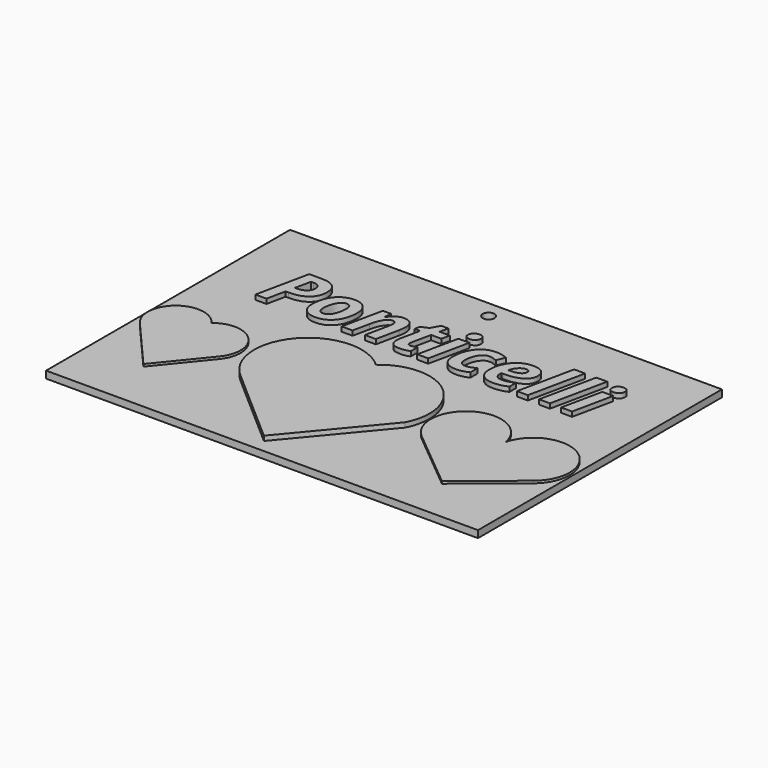
from build123d import *

# Parameters (mm, degrees)
F0_TEXT_SIZE = 31.6076549805
F1_DEPTH     = 5
F0_W         = 183.1867024302
F0_H         = 129.334770143
F2_DEPTH     = 3
F4_DEPTH     = 1
F5_D         = 5


# Not quite as in the source:
# - Text() gives the source's letters only with a copy of the font that has no kerning and outlines rounded to 1/6400 em; it was checked with that copy


with BuildPart() as f1:
    # F0 (on Top) → F1 (new body)
    with BuildSketch(Plane.XY):
        with Locations((-77.6233896613, 8.2242488861)):
            Text('Ponticelli', F0_TEXT_SIZE, font='Open Sans', font_style=FontStyle.BOLDITALIC, text_align=(TextAlign.LEFT, TextAlign.BOTTOM))
        with BuildLine():
            ThreePointArc((19.1414519703, -32.36814572), (13.3379238133, -5.4645873951), (-14.1757235594, -6.1585599173))
            ThreePointArc((-14.1757235594, -6.1585599173), (-46.727283961, -7.8440457742), (-44.2183457938, -40.3425099906))
            Line((-44.2183457938, -40.3425099906), (-11.378755793, -69.0611600876))
            Line((-11.378755793, -69.0611600876), (19.1414519703, -32.36814572))
        make_face()
    extrude(amount=F1_DEPTH)

    # F0 (on Top) → F2 (join)
    with BuildSketch(Plane.XY):
        with Locations((-7.6609440148, -10.0268237293)):
            Rectangle(F0_W, F0_H)
        with BuildLine():
            ThreePointArc((-44.2183457938, -40.3425099906), (-46.727283961, -7.8440457742), (-14.1757235594, -6.1585599173))
            ThreePointArc((-14.1757235594, -6.1585599173), (13.3379238133, -5.4645873951), (19.1414519703, -32.36814572))
            Line((19.1414519703, -32.36814572), (-11.378755793, -69.0611600876))
            Line((-11.378755793, -69.0611600876), (-44.2183457938, -40.3425099906))
        make_face(mode=Mode.SUBTRACT)
        with BuildLine():
            add(Edge.make_bspline(
                [(-61.1701236351, 29.1445655263), (-59.2563789, 27.4999797281), (-59.2563789, 24.2157468278)],
                knots=[0, 0, 0, 1, 1, 1], degree=2))
            add(Edge.make_bspline(
                [(-59.2563789, 24.2157468278), (-59.2563789, 20.4919699754), (-61.8738878281, 18.3708000045)],
                knots=[0, 0, 0, 1, 1, 1], degree=2))
            add(Edge.make_bspline(
                [(-61.8738878281, 18.3708000045), (-64.4913967561, 16.2496300335), (-69.0893228166, 16.2496300335)],
                knots=[0, 0, 0, 1, 1, 1], degree=2))
            Line((-69.0893228166, 16.2496300335), (-70.417832065, 16.2496300335))
            Line((-70.417832065, 16.2496300335), (-72.0969887358, 8.2242488861))
            Line((-72.0969887358, 8.2242488861), (-76.8035661103, 8.2242488861))
            Line((-76.8035661103, 8.2242488861), (-72.0377243827, 30.7891513245))
            Line((-72.0377243827, 30.7891513245), (-66.8175226149, 30.7891513245))
            add(Edge.make_bspline(
                [(-66.8175226149, 30.7891513245), (-63.0838683703, 30.7891513245), (-61.1701236351, 29.1445655263)],
                knots=[0, 0, 0, 1, 1, 1], degree=2))
        make_face(mode=Mode.SUBTRACT)
        with BuildLine():
            add(Edge.make_bspline(
                [(-43.9439516708, 23.9811587635), (-42.1833065144, 22.1612492541), (-42.1833065144, 18.9659128834)],
                knots=[0, 0, 0, 1, 1, 1], degree=2))
            add(Edge.make_bspline(
                [(-42.1833065144, 18.9659128834), (-42.1833065144, 15.7113121596), (-43.2722890024, 13.1950465014)],
                knots=[0, 0, 0, 1, 1, 1], degree=2))
            add(Edge.make_bspline(
                [(-43.2722890024, 13.1950465014), (-44.3612714904, 10.6787808432), (-46.4132997161, 9.2959459378)],
                knots=[0, 0, 0, 1, 1, 1], degree=2))
            add(Edge.make_bspline(
                [(-46.4132997161, 9.2959459378), (-48.4653279418, 7.9131110324), (-51.2902621057, 7.9131110324)],
                knots=[0, 0, 0, 1, 1, 1], degree=2))
            add(Edge.make_bspline(
                [(-51.2902621057, 7.9131110324), (-54.302866721, 7.9131110324), (-56.100552098, 9.7280818457)],
                knots=[0, 0, 0, 1, 1, 1], degree=2))
            add(Edge.make_bspline(
                [(-56.100552098, 9.7280818457), (-57.8982374751, 11.5430526591), (-57.8982374751, 14.5507185783)],
                knots=[0, 0, 0, 1, 1, 1], degree=2))
            add(Edge.make_bspline(
                [(-57.8982374751, 14.5507185783), (-57.8982374751, 17.8398901747), (-56.7944388988, 20.4104814899)],
                knots=[0, 0, 0, 1, 1, 1], degree=2))
            add(Edge.make_bspline(
                [(-56.7944388988, 20.4104814899), (-55.6906403225, 22.9810728051), (-53.6065105722, 24.391070539)],
                knots=[0, 0, 0, 1, 1, 1], degree=2))
            add(Edge.make_bspline(
                [(-53.6065105722, 24.391070539), (-51.522380822, 25.8010682729), (-48.7270788346, 25.8010682729)],
                knots=[0, 0, 0, 1, 1, 1], degree=2))
            add(Edge.make_bspline(
                [(-48.7270788346, 25.8010682729), (-45.7045968271, 25.8010682729), (-43.9439516708, 23.9811587635)],
                knots=[0, 0, 0, 1, 1, 1], degree=2))
        make_face(mode=Mode.SUBTRACT)
        with BuildLine():
            Line((-23.6631961743, 18.0571928027), (-25.717693748, 8.2242488861))
            Line((-25.717693748, 8.2242488861), (-30.3600680733, 8.2242488861))
            Line((-30.3600680733, 8.2242488861), (-28.2463061465, 18.3041276072))
            add(Edge.make_bspline(
                [(-28.2463061465, 18.3041276072), (-27.9993713419, 19.3511311785), (-27.9993713419, 20.141322553)],
                knots=[0, 0, 0, 1, 1, 1], degree=2))
            add(Edge.make_bspline(
                [(-27.9993713419, 20.141322553), (-27.9993713419, 22.0377818518), (-29.6686506206, 22.0377818518)],
                knots=[0, 0, 0, 1, 1, 1], degree=2))
            add(Edge.make_bspline(
                [(-29.6686506206, 22.0377818518), (-31.0860563986, 22.0377818518), (-32.2441806319, 20.2771366955)],
                knots=[0, 0, 0, 1, 1, 1], degree=2))
            add(Edge.make_bspline(
                [(-32.2441806319, 20.2771366955), (-33.4023048652, 18.5164915391), (-34.0640901413, 15.3705421294)],
                knots=[0, 0, 0, 1, 1, 1], degree=2))
            Line((-34.0640901413, 15.3705421294), (-35.5802698412, 8.2242488861))
            Line((-35.5802698412, 8.2242488861), (-40.2226441664, 8.2242488861))
            Line((-40.2226441664, 8.2242488861), (-36.5680090593, 25.480053027))
            Line((-36.5680090593, 25.480053027), (-33.0170865701, 25.480053027))
            Line((-33.0170865701, 25.480053027), (-33.3430405121, 22.2847166563))
            Line((-33.3430405121, 22.2847166563), (-33.2492052864, 22.2847166563))
            add(Edge.make_bspline(
                [(-33.2492052864, 22.2847166563), (-30.997159869, 25.8010682729), (-27.7672526257, 25.8010682729)],
                knots=[0, 0, 0, 1, 1, 1], degree=2))
            add(Edge.make_bspline(
                [(-27.7672526257, 25.8010682729), (-25.6386746106, 25.8010682729), (-24.4731423332, 24.5145379413)],
                knots=[0, 0, 0, 1, 1, 1], degree=2))
            add(Edge.make_bspline(
                [(-24.4731423332, 24.5145379413), (-23.3076100558, 23.2280076097), (-23.3076100558, 20.8327400057)],
                knots=[0, 0, 0, 1, 1, 1], degree=2))
            add(Edge.make_bspline(
                [(-23.3076100558, 20.8327400057), (-23.3076100558, 19.706717297), (-23.6631961743, 18.0571928027)],
                knots=[0, 0, 0, 1, 1, 1], degree=2))
        make_face(mode=Mode.SUBTRACT)
        with BuildLine():
            add(Edge.make_bspline(
                [(-15.1291293296, 12.8073588583), (-15.1291293296, 11.6665200613), (-13.7709879046, 11.6665200613)],
                knots=[0, 0, 0, 1, 1, 1], degree=2))
            add(Edge.make_bspline(
                [(-13.7709879046, 11.6665200613), (-12.7684325982, 11.6665200613), (-11.2670689867, 12.2048379352)],
                knots=[0, 0, 0, 1, 1, 1], degree=2))
            Line((-11.2670689867, 12.2048379352), (-11.2670689867, 8.7329345835))
            add(Edge.make_bspline(
                [(-11.2670689867, 8.7329345835), (-12.9807965301, 7.9131110324), (-15.3760641341, 7.9131110324)],
                knots=[0, 0, 0, 1, 1, 1], degree=2))
            add(Edge.make_bspline(
                [(-15.3760641341, 7.9131110324), (-17.6873739046, 7.9131110324), (-18.7763563926, 8.8860341623)],
                knots=[0, 0, 0, 1, 1, 1], degree=2))
            add(Edge.make_bspline(
                [(-18.7763563926, 8.8860341623), (-19.8653388806, 9.8589572921), (-19.8653388806, 11.8986387776)],
                knots=[0, 0, 0, 1, 1, 1], degree=2))
            add(Edge.make_bspline(
                [(-19.8653388806, 11.8986387776), (-19.8653388806, 12.6690753677), (-19.6826071252, 13.6271824093)],
                knots=[0, 0, 0, 1, 1, 1], degree=2))
            Line((-19.6826071252, 13.6271824093), (-17.9046765326, 21.9439466261))
            Line((-17.9046765326, 21.9439466261), (-20.2505571756, 21.9439466261))
            Line((-20.2505571756, 21.9439466261), (-19.8060745275, 24.2157468278))
            Line((-19.8060745275, 24.2157468278), (-16.7786538239, 25.5096852036))
            Line((-16.7786538239, 25.5096852036), (-14.7439110345, 29.1544429185))
            Line((-14.7439110345, 29.1544429185), (-11.7461225074, 29.1544429185))
            Line((-11.7461225074, 29.1544429185), (-12.5017430093, 25.480053027))
            Line((-12.5017430093, 25.480053027), (-8.1359356651, 25.480053027))
            Line((-8.1359356651, 25.480053027), (-8.9063722553, 21.9439466261))
            Line((-8.9063722553, 21.9439466261), (-13.2623022073, 21.9439466261))
            Line((-13.2623022073, 21.9439466261), (-15.0352941039, 13.6271824093))
            add(Edge.make_bspline(
                [(-15.0352941039, 13.6271824093), (-15.1291293296, 13.1629449768), (-15.1291293296, 12.8073588583)],
                knots=[0, 0, 0, 1, 1, 1], degree=2))
        make_face(mode=Mode.SUBTRACT)
        Polygon((0.1363802868, 25.480053027), (-3.5231935164, 8.2242488861), (-8.1655678417, 8.2242488861), (-4.5109327346, 25.480053027), align=None, mode=Mode.SUBTRACT)
        with BuildLine():
            add(Edge.make_bspline(
                [(13.6387753988, 9.1329689668), (11.2928947557, 7.9131110324), (8.4531445035, 7.9131110324)],
                knots=[0, 0, 0, 1, 1, 1], degree=2))
            add(Edge.make_bspline(
                [(8.4531445035, 7.9131110324), (5.3516433586, 7.9131110324), (3.6922414721, 9.5725129189)],
                knots=[0, 0, 0, 1, 1, 1], degree=2))
            add(Edge.make_bspline(
                [(3.6922414721, 9.5725129189), (2.0328395856, 11.2319148053), (2.0328395856, 14.2593355089)],
                knots=[0, 0, 0, 1, 1, 1], degree=2))
            add(Edge.make_bspline(
                [(2.0328395856, 14.2593355089), (2.0328395856, 17.528752321), (3.1835557747, 20.2079949502)],
                knots=[0, 0, 0, 1, 1, 1], degree=2))
            add(Edge.make_bspline(
                [(3.1835557747, 20.2079949502), (4.3342719639, 22.8872375794), (6.4184017141, 24.3441529262)],
                knots=[0, 0, 0, 1, 1, 1], degree=2))
            add(Edge.make_bspline(
                [(6.4184017141, 24.3441529262), (8.5025314644, 25.8010682729), (11.1694273534, 25.8010682729)],
                knots=[0, 0, 0, 1, 1, 1], degree=2))
            add(Edge.make_bspline(
                [(11.1694273534, 25.8010682729), (13.979545429, 25.8010682729), (16.2315908464, 24.6898616525)],
                knots=[0, 0, 0, 1, 1, 1], degree=2))
            Line((16.2315908464, 24.6898616525), (14.8141850683, 21.1586939477))
            add(Edge.make_bspline(
                [(14.8141850683, 21.1586939477), (13.979545429, 21.5142800662), (13.1770073143, 21.776030959)],
                knots=[0, 0, 0, 1, 1, 1], degree=2))
            add(Edge.make_bspline(
                [(13.1770073143, 21.776030959), (12.3744691995, 22.0377818518), (11.3570978049, 22.0377818518)],
                knots=[0, 0, 0, 1, 1, 1], degree=2))
            add(Edge.make_bspline(
                [(11.3570978049, 22.0377818518), (10.0434046447, 22.0377818518), (8.9865236813, 21.0500426337)],
                knots=[0, 0, 0, 1, 1, 1], degree=2))
            add(Edge.make_bspline(
                [(8.9865236813, 21.0500426337), (7.9296427179, 20.0623034155), (7.334529839, 18.3411678279)],
                knots=[0, 0, 0, 1, 1, 1], degree=2))
            add(Edge.make_bspline(
                [(7.334529839, 18.3411678279), (6.73941696, 16.6200322403), (6.73941696, 14.644553804)],
                knots=[0, 0, 0, 1, 1, 1], degree=2))
            add(Edge.make_bspline(
                [(6.73941696, 14.644553804), (6.73941696, 13.1629449768), (7.443181153, 12.4147325191)],
                knots=[0, 0, 0, 1, 1, 1], degree=2))
            add(Edge.make_bspline(
                [(7.443181153, 12.4147325191), (8.1469453459, 11.6665200613), (9.3964354568, 11.6665200613)],
                knots=[0, 0, 0, 1, 1, 1], degree=2))
            add(Edge.make_bspline(
                [(9.3964354568, 11.6665200613), (10.5669064303, 11.6665200613), (11.5719310848, 12.029514224)],
                knots=[0, 0, 0, 1, 1, 1], degree=2))
            add(Edge.make_bspline(
                [(11.5719310848, 12.029514224), (12.5769557393, 12.3925083867), (13.6387753988, 12.9308262605)],
                knots=[0, 0, 0, 1, 1, 1], degree=2))
            Line((13.6387753988, 12.9308262605), (13.6387753988, 9.1329689668))
        make_face(mode=Mode.SUBTRACT)
        with BuildLine():
            add(Edge.make_bspline(
                [(30.1389590378, 9.2416202808), (27.4868792371, 7.9131110324), (24.1236271993, 7.9131110324)],
                knots=[0, 0, 0, 1, 1, 1], degree=2))
            add(Edge.make_bspline(
                [(24.1236271993, 7.9131110324), (20.8789038677, 7.9131110324), (19.0886265348, 9.6589401005)],
                knots=[0, 0, 0, 1, 1, 1], degree=2))
            add(Edge.make_bspline(
                [(19.0886265348, 9.6589401005), (17.298349202, 11.4047691685), (17.298349202, 14.5852894509)],
                knots=[0, 0, 0, 1, 1, 1], degree=2))
            add(Edge.make_bspline(
                [(17.298349202, 14.5852894509), (17.298349202, 17.7756871255), (18.5725327934, 20.4080121419)],
                knots=[0, 0, 0, 1, 1, 1], degree=2))
            add(Edge.make_bspline(
                [(18.5725327934, 20.4080121419), (19.8467163848, 23.0403371582), (22.0222120127, 24.4207027156)],
                knots=[0, 0, 0, 1, 1, 1], degree=2))
            add(Edge.make_bspline(
                [(22.0222120127, 24.4207027156), (24.1977076407, 25.8010682729), (26.9436226671, 25.8010682729)],
                knots=[0, 0, 0, 1, 1, 1], degree=2))
            add(Edge.make_bspline(
                [(26.9436226671, 25.8010682729), (29.6796603014, 25.8010682729), (31.2057173934, 24.5441701178)],
                knots=[0, 0, 0, 1, 1, 1], degree=2))
            add(Edge.make_bspline(
                [(31.2057173934, 24.5441701178), (32.7317744854, 23.2872719627), (32.7317744854, 21.0944908985)],
                knots=[0, 0, 0, 1, 1, 1], degree=2))
            add(Edge.make_bspline(
                [(32.7317744854, 21.0944908985), (32.7317744854, 18.2102923815), (30.1562444741, 16.6447257208)],
                knots=[0, 0, 0, 1, 1, 1], degree=2))
            add(Edge.make_bspline(
                [(30.1562444741, 16.6447257208), (27.5807144628, 15.07915906), (22.7951179509, 15.07915906)],
                knots=[0, 0, 0, 1, 1, 1], degree=2))
            Line((22.7951179509, 15.07915906), (22.0049265764, 15.07915906))
            Line((22.0049265764, 15.07915906), (21.9752943999, 14.753205118))
            Line((21.9752943999, 14.753205118), (21.9752943999, 14.4420672643))
            add(Edge.make_bspline(
                [(21.9752943999, 14.4420672643), (21.9752943999, 13.0394775745), (22.7704244705, 12.2295314157)],
                knots=[0, 0, 0, 1, 1, 1], degree=2))
            add(Edge.make_bspline(
                [(22.7704244705, 12.2295314157), (23.5655545411, 11.4195852568), (25.0471633683, 11.4195852568)],
                knots=[0, 0, 0, 1, 1, 1], degree=2))
            add(Edge.make_bspline(
                [(25.0471633683, 11.4195852568), (26.3904887049, 11.4195852568), (27.4868792371, 11.7134376742)],
                knots=[0, 0, 0, 1, 1, 1], degree=2))
            add(Edge.make_bspline(
                [(27.4868792371, 11.7134376742), (28.5832697692, 12.0072900916), (30.1389590378, 12.7480945052)],
                knots=[0, 0, 0, 1, 1, 1], degree=2))
            Line((30.1389590378, 12.7480945052), (30.1389590378, 9.2416202808))
        make_face(mode=Mode.SUBTRACT)
        Polygon((43.8339632973, 32.2411279752), (38.7372289317, 8.2242488861), (34.0948546064, 8.2242488861), (39.186650276, 32.2411279752), align=None, mode=Mode.SUBTRACT)
        Polygon((53.2174858696, 32.2411279752), (48.120751504, 8.2242488861), (43.4783771788, 8.2242488861), (48.5701728483, 32.2411279752), align=None, mode=Mode.SUBTRACT)
        Polygon((61.1638478796, 25.480053027), (57.5042740764, 8.2242488861), (52.8618997511, 8.2242488861), (56.5165348582, 25.480053027), align=None, mode=Mode.SUBTRACT)
        with BuildLine():
            add(Edge.make_bspline(
                [(-1.4390637662, 27.6234471304), (-3.770128321, 27.6234471304), (-3.770128321, 29.5248451253)],
                knots=[0, 0, 0, 1, 1, 1], degree=2))
            add(Edge.make_bspline(
                [(-3.770128321, 29.5248451253), (-3.770128321, 30.8632317659), (-3.0367319515, 31.5521798705)],
                knots=[0, 0, 0, 1, 1, 1], degree=2))
            add(Edge.make_bspline(
                [(-3.0367319515, 31.5521798705), (-2.303335582, 32.2411279752), (-0.9600102454, 32.2411279752)],
                knots=[0, 0, 0, 1, 1, 1], degree=2))
            add(Edge.make_bspline(
                [(-0.9600102454, 32.2411279752), (0.1660124633, 32.2411279752), (0.7537172981, 31.7620744544)],
                knots=[0, 0, 0, 1, 1, 1], degree=2))
            add(Edge.make_bspline(
                [(0.7537172981, 31.7620744544), (1.3414221329, 31.2830209336), (1.3414221329, 30.3891169412)],
                knots=[0, 0, 0, 1, 1, 1], degree=2))
            add(Edge.make_bspline(
                [(1.3414221329, 30.3891169412), (1.3414221329, 29.1544429185), (0.6623514204, 28.3889450244)],
                knots=[0, 0, 0, 1, 1, 1], degree=2))
            add(Edge.make_bspline(
                [(0.6623514204, 28.3889450244), (-0.016719292, 27.6234471304), (-1.4390637662, 27.6234471304)],
                knots=[0, 0, 0, 1, 1, 1], degree=2))
        make_face(mode=Mode.SUBTRACT)
        with BuildLine():
            add(Edge.make_bspline(
                [(59.5884038266, 27.6234471304), (57.2573392718, 27.6234471304), (57.2573392718, 29.5248451253)],
                knots=[0, 0, 0, 1, 1, 1], degree=2))
            add(Edge.make_bspline(
                [(57.2573392718, 29.5248451253), (57.2573392718, 30.8632317659), (57.9907356413, 31.5521798705)],
                knots=[0, 0, 0, 1, 1, 1], degree=2))
            add(Edge.make_bspline(
                [(57.9907356413, 31.5521798705), (58.7241320108, 32.2411279752), (60.0674573474, 32.2411279752)],
                knots=[0, 0, 0, 1, 1, 1], degree=2))
            add(Edge.make_bspline(
                [(60.0674573474, 32.2411279752), (61.1934800561, 32.2411279752), (61.7811848909, 31.7620744544)],
                knots=[0, 0, 0, 1, 1, 1], degree=2))
            add(Edge.make_bspline(
                [(61.7811848909, 31.7620744544), (62.3688897257, 31.2830209336), (62.3688897257, 30.3891169412)],
                knots=[0, 0, 0, 1, 1, 1], degree=2))
            add(Edge.make_bspline(
                [(62.3688897257, 30.3891169412), (62.3688897257, 29.1544429185), (61.6898190132, 28.3889450244)],
                knots=[0, 0, 0, 1, 1, 1], degree=2))
            add(Edge.make_bspline(
                [(61.6898190132, 28.3889450244), (61.0107483008, 27.6234471304), (59.5884038266, 27.6234471304)],
                knots=[0, 0, 0, 1, 1, 1], degree=2))
        make_face(mode=Mode.SUBTRACT)
    extrude(amount=F2_DEPTH)

    # F3 (on face) → F4 (join)
    with BuildSketch(Plane.XY.offset(3)):
        with BuildLine():
            ThreePointArc((-59.5361028212, -32.2895134146), (-60.3734979534, -16.0705564952), (-76.5933134618, -15.249959741))
            ThreePointArc((-76.5933134618, -15.249959741), (-93.6287776466, -12.9097233176), (-95.2184288727, -30.0315443507))
            Line((-95.2184288727, -30.0315443507), (-75.8489966393, -52.3492991924))
            Line((-75.8489966393, -52.3492991924), (-59.5361028212, -32.2895134146))
        make_face()
        with BuildLine():
            Line((53.8279563189, -56.1720430851), (77.3787288939, -36.9470299717))
            ThreePointArc((77.3787288939, -36.9470299717), (76.0054454376, -12.0927944135), (52.7723430212, -21.02822304))
            ThreePointArc((52.7723430212, -21.02822304), (30.5005274664, -10.8829870359), (28.5581053765, -35.2794330498))
            Line((28.5581053765, -35.2794330498), (53.8279563189, -56.1720430851))
        make_face()
    extrude(amount=F4_DEPTH)

    # F5 (through all)
    with Locations(Plane.XY.offset(3)):
        with Locations((-9.2381965369, 47.4302582443)):
            Hole(F5_D / 2)


solid = f1.part
